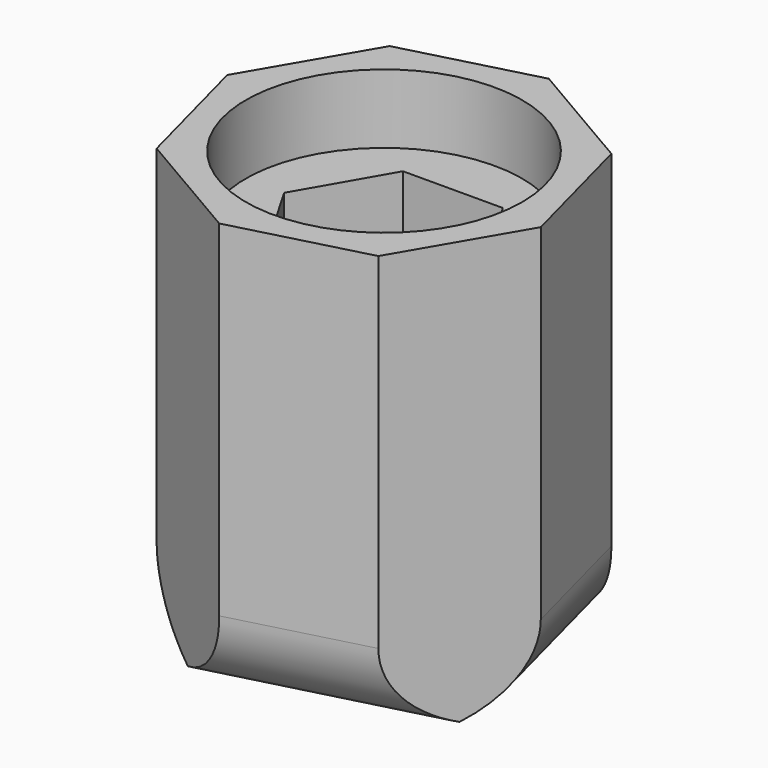
from build123d import *

# Parameters (mm, degrees)
F0_R        = 8
F1_DEPTH    = 20
F0_R_2      = 3
F2_DEPTH    = 5
F3_DEPTH    = 10
F4_DEPTH    = 16
F5_T1_DEPTH = 32.8700576851
F5_T3_DEPTH = 32.8700576851
F5_T5_DEPTH = 32.8700576851
F5_T7_DEPTH = 32.8700576851


# Not quite as in the source:
# - a fillet or chamfer that OpenCascade refuses, or shapes differently, is made with other operations: its cross-section is extruded or revolved along the edge and cut away or added


with BuildPart() as f1:
    # F0 (on Top) → F1 (new body)
    with BuildSketch(Plane.XY):
        Polygon((6.2218713056, -8.1867435191), (10.1884292501, -1.3893744663), (8.1867435191, 6.2218713056), (1.3893744663, 10.1884292501), (-6.2218713056, 8.1867435191), (-10.1884292501, 1.3893744663), (-8.1867435191, -6.2218713056), (-1.3893744663, -10.1884292501), align=None)
        Circle(F0_R, mode=Mode.SUBTRACT)
    extrude(amount=F1_DEPTH)

    # F0 (on Top) → F2 (join)
    with BuildSketch(Plane.XY):
        Polygon((6.2218713056, -8.1867435191), (10.1884292501, -1.3893744663), (8.1867435191, 6.2218713056), (1.3893744663, 10.1884292501), (-6.2218713056, 8.1867435191), (-10.1884292501, 1.3893744663), (-8.1867435191, -6.2218713056), (-1.3893744663, -10.1884292501), align=None)
        Circle(F0_R, mode=Mode.SUBTRACT)
        Circle(F0_R)
        Polygon((-2.8984208181, 4.9932444457), (2.8750661283, 5.0067282822), (5.7734869463, 0.0134838364), (2.8984208181, -4.9932444457), (-2.8750661283, -5.0067282822), (-5.7734869463, -0.0134838364), align=None, mode=Mode.SUBTRACT)
        Polygon((5.7734869463, 0.0134838364), (2.8750661283, 5.0067282822), (-2.8984208181, 4.9932444457), (-5.7734869463, -0.0134838364), (-2.8750661283, -5.0067282822), (2.8984208181, -4.9932444457), align=None)
        Circle(F0_R_2, mode=Mode.SUBTRACT)
        Circle(F0_R_2)
    extrude(amount=-F2_DEPTH)

    # F0 (on Top) → F3 (join)
    with BuildSketch(Plane.XY):
        Polygon((5.7734869463, 0.0134838364), (2.8750661283, 5.0067282822), (-2.8984208181, 4.9932444457), (-5.7734869463, -0.0134838364), (-2.8750661283, -5.0067282822), (2.8984208181, -4.9932444457), align=None)
        Circle(F0_R_2, mode=Mode.SUBTRACT)
    extrude(amount=F3_DEPTH)

    # F5: fillet of radius 5 on 4 edges, made by hand

    # F5_s2 → F5_t1 (cut)
    with BuildSketch(Plane(origin=(-15.8945523394, -4.1801171018, 0), x_dir=(0, 0, 1), z_dir=(0.9671143563, 0.2543419389, 0))):
        with BuildLine():
            ThreePointArc((0, 9.5), (-3.5355339059, 8.0355339059), (-5, 4.5))
            Line((-5, 4.5), (-5, 9.5))
            Line((-5, 9.5), (0, 9.5))
        make_face()
    extrude(amount=F5_T1_DEPTH, mode=Mode.SUBTRACT)

    # F5_s4 → F5_t3 (cut)
    with BuildSketch(Plane(origin=(-4.1801171018, 15.8945523394, 0), x_dir=(0, 0, 1), z_dir=(0.2543419389, -0.9671143563, 0))):
        with BuildLine():
            ThreePointArc((0, 9.5), (-3.5355339059, 8.0355339059), (-5, 4.5))
            Line((-5, 4.5), (-5, 9.5))
            Line((-5, 9.5), (0, 9.5))
        make_face()
    extrude(amount=F5_T3_DEPTH, mode=Mode.SUBTRACT)

    # F5_s6 → F5_t5 (cut)
    with BuildSketch(Plane(origin=(15.8945523394, 4.1801171018, 0), x_dir=(0, 0, 1), z_dir=(-0.9671143563, -0.2543419389, 0))):
        with BuildLine():
            ThreePointArc((-5, 4.5), (-3.5355339059, 8.0355339059), (0, 9.5))
            Line((0, 9.5), (-5, 9.5))
            Line((-5, 9.5), (-5, 4.5))
        make_face()
    extrude(amount=F5_T5_DEPTH, mode=Mode.SUBTRACT)

    # F5_s8 → F5_t7 (cut)
    with BuildSketch(Plane(origin=(4.1801171018, -15.8945523394, 0), x_dir=(0, 0, 1), z_dir=(-0.2543419389, 0.9671143563, 0))):
        with BuildLine():
            ThreePointArc((-5, 4.5), (-3.5355339059, 8.0355339059), (0, 9.5))
            Line((0, 9.5), (-5, 9.5))
            Line((-5, 9.5), (-5, 4.5))
        make_face()
    extrude(amount=F5_T7_DEPTH, mode=Mode.SUBTRACT)


with BuildPart() as f4:
    # F0 (on Top) → F4 (new body)
    with BuildSketch(Plane.XY):
        Circle(F0_R)
        Polygon((-2.8984208181, 4.9932444457), (2.8750661283, 5.0067282822), (5.7734869463, 0.0134838364), (2.8984208181, -4.9932444457), (-2.8750661283, -5.0067282822), (-5.7734869463, -0.0134838364), align=None, mode=Mode.SUBTRACT)
    extrude(amount=F4_DEPTH)


solid = Compound([f1.part, f4.part])
